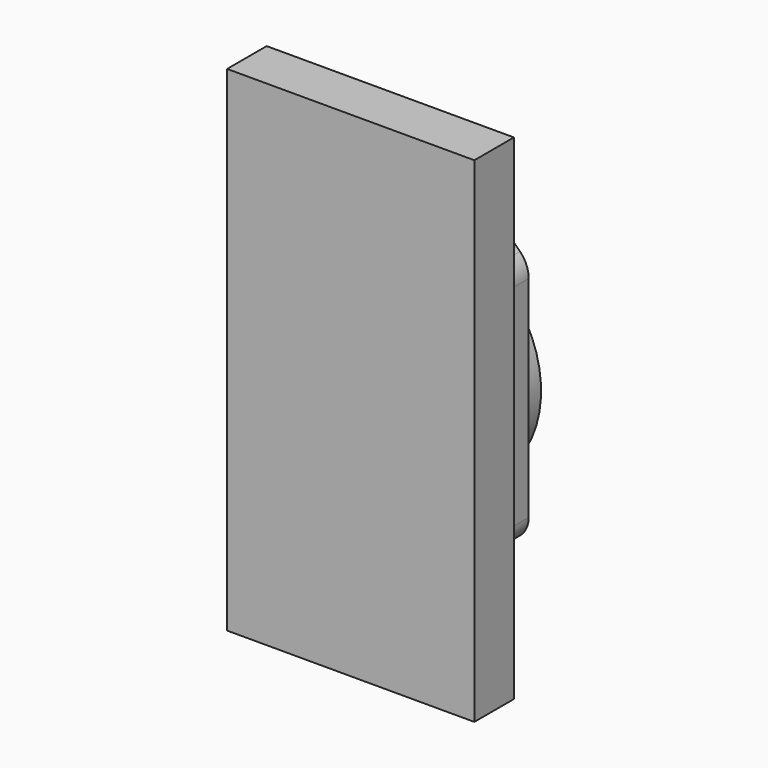
from build123d import *

# Parameters (mm, degrees)
F0_W     = 100
F0_H     = 200
F1_DEPTH = 20
F3_DEPTH = 15
F2_R     = 45
F4_DEPTH = 10
F2_R_2   = 5
F2_R_3   = 30
F5_DEPTH = 20
F6_D     = 10
F6_DEPTH = 15
F6_TIP   = 3.0043030951
F7_DEPTH = 12


with BuildPart() as f1:
    # F0 (on Front) → F1 (new body)
    with BuildSketch(Plane.XZ):
        Rectangle(F0_W, F0_H)
    extrude(amount=F1_DEPTH)

    # F2 (on face) → F3 (cut)
    with BuildSketch(Plane(origin=(0, 0, 0), x_dir=(-1, 0, 0), z_dir=(0, 1, 0))):
        with BuildLine():
            ThreePointArc((-40, -78), (-36.4852813742, -86.4852813742), (-28, -90))
            Line((-28, -90), (28, -90))
            ThreePointArc((28, -90), (36.4852813742, -86.4852813742), (40, -78))
            Line((40, -78), (40, -72))
            ThreePointArc((40, -72), (36.4852813742, -63.5147186258), (28, -60))
            Line((28, -60), (-28, -60))
            ThreePointArc((-28, -60), (-36.4852813742, -63.5147186258), (-40, -72))
            Line((-40, -72), (-40, -78))
        make_face()
    extrude(amount=-F3_DEPTH, mode=Mode.SUBTRACT)

    # F6
    with Locations(Plane(origin=(0, 0, 0), x_dir=(-1, 0, 0), z_dir=(0, 1, 0))):
        with Locations((-37.5, 0), (0, -37.5), (37.5, 0), (0, 37.5)):
            Hole(F6_D / 2, depth=F6_DEPTH)
            with Locations((0, 0, -(F6_DEPTH + F6_TIP / 2))):  # 118° drill point
                Cone(0, F6_D / 2, F6_TIP, mode=Mode.SUBTRACT)

    # F2 (on face) → F7 (cut)
    with BuildSketch(Plane(origin=(0, 0, 0), x_dir=(-1, 0, 0), z_dir=(0, 1, 0))):
        Circle(F2_R_3)
    extrude(amount=-F7_DEPTH, mode=Mode.SUBTRACT)


with BuildPart() as f4:
    # F2 (on face) → F4 (new body)
    with BuildSketch(Plane(origin=(0, 0, 0), x_dir=(-1, 0, 0), z_dir=(0, 1, 0))):
        with BuildLine():
            ThreePointArc((-48, -40), (-45.0710678119, -47.0710678119), (-38, -50))
            Line((-38, -50), (38, -50))
            ThreePointArc((38, -50), (45.0710678119, -47.0710678119), (48, -40))
            Line((48, -40), (48, 45.029))
            ThreePointArc((48, 45.029), (47.0866406093, 49.6209930314), (44.4856, 53.5139627365))
            Line((44.4856, 53.5139627365), (10.607, 87.3951071902))
            ThreePointArc((10.607, 87.3951071902), (0, 91.7889037696), (-10.607, 87.3951071902))
            Line((-10.607, 87.3951071902), (-44.4856, 53.5139627365))
            ThreePointArc((-44.4856, 53.5139627365), (-47.0866406093, 49.6209930314), (-48, 45.029))
            Line((-48, 45.029), (-48, -40))
        make_face()
        Circle(F2_R, mode=Mode.SUBTRACT)
    extrude(amount=F4_DEPTH)


with BuildPart() as f5:
    # F2 (on face) → F5 (new body)
    with BuildSketch(Plane(origin=(0, 0, 0), x_dir=(-1, 0, 0), z_dir=(0, 1, 0))):
        Circle(F2_R)
        with Locations((0, -37.5)):
            Circle(F2_R_2, mode=Mode.SUBTRACT)
        with Locations((-37.5, 0)):
            Circle(F2_R_2, mode=Mode.SUBTRACT)
        Circle(F2_R_3, mode=Mode.SUBTRACT)
        with Locations((0, 37.5)):
            Circle(F2_R_2, mode=Mode.SUBTRACT)
        with Locations((37.5, 0)):
            Circle(F2_R_2, mode=Mode.SUBTRACT)
    extrude(amount=F5_DEPTH)


solid = Compound([f1.part, f4.part, f5.part])
